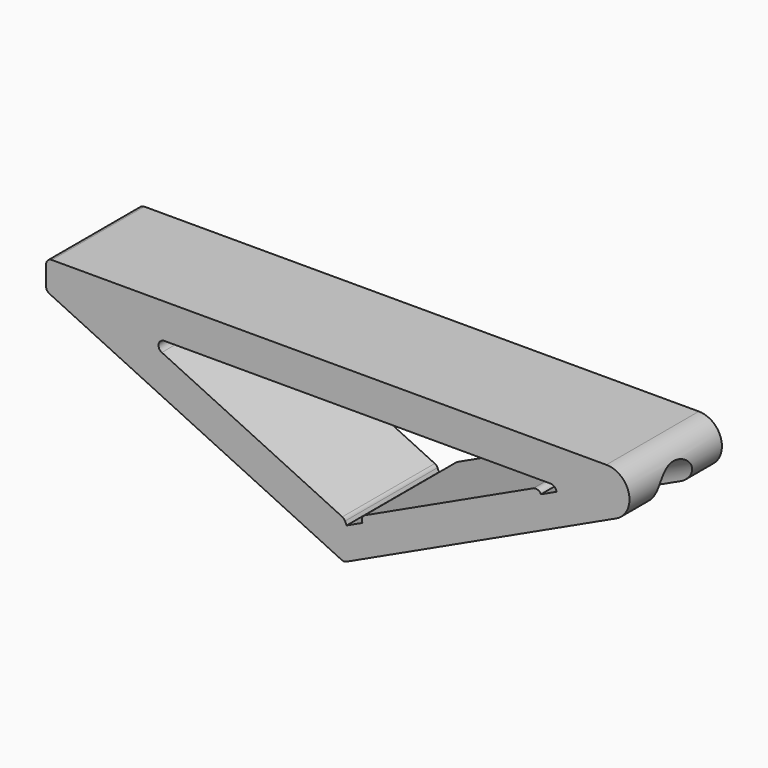
from build123d import *

# Parameters (mm, degrees)
F1_DEPTH  = 50
F3_R      = 1
F4_R      = 4
F5_R      = 4
F6_DEPTH  = 116.6842043143
F8_DEPTH  = 50.0010001
F9_R      = 0.99999
F10_DEPTH = 30


# Not quite as in the source:
# - a fillet or chamfer is up to 0.001 mm smaller than in the source, because OpenCascade refuses the exact size


with BuildPart() as f1:
    # F0 (on Front) → F1 (new body)
    with BuildSketch(Plane.XZ):
        Polygon((-63.4415450926, -29.5832783218), (0, 0), (-115, 0), (-115, -5), align=None)
    extrude(amount=F1_DEPTH)

    # F3
    f3_edges = [f1.edges().sort_by_distance(p)[0] for p in [
        (-63.441545, -25, -29.583278),
        (-115, -25, -5),
        (-115, -25, 0),
    ]]
    fillet(f3_edges, radius=F3_R)

    # F4
    f4_edges = [f1.edges().sort_by_distance(p)[0] for p in [
        (0, -25, 0),
    ]]
    fillet(f4_edges, radius=F4_R)

    # F5 (on face) → F6 (cut, through all)
    with BuildSketch(Plane(origin=(0, 0, 0), x_dir=(0, 1, 0), z_dir=(0.906307787, 0, 0.4226182617))):
        with Locations((-40, 0)):
            Circle(F5_R)
    extrude(amount=-F6_DEPTH, mode=Mode.SUBTRACT)

    # F7 (on Front) → F8 (cut, through all)
    with BuildSketch(Plane.XZ):
        Polygon((-27.064251022, -6), (-98.9616948614, -6), (-63.4130640807, -22.9497298941), (-62.990445819, -23.8560376812), (-60.2715224579, -22.588182896), (-60.6941407196, -21.6818751089), (-29.7831743831, -7.2678547852), (-29.3605561213, -8.1741625723), (-26.6416327602, -6.906307787), align=None)
    extrude(amount=F8_DEPTH, mode=Mode.SUBTRACT)

    # F9 (radius 1 in the source; OpenCascade refuses exactly that, so slightly less here)
    f9_edges = [f1.edges().sort_by_distance(p)[0] for p in [
        (-98.961695, -25, -6),
        (-60.694141, -25, -21.681875),
        (-29.783174, -25, -7.267855),
        (-27.064251, -25, -6),
        (-63.413064, -25, -22.94973),
    ]]
    fillet(f9_edges, radius=F9_R)

    # F0 (on Front) → F10 (cut)
    with BuildSketch(Plane.XZ):
        Polygon((-63.4415450926, -29.5832783218), (0, 0), (-115, 0), (-115, -5), align=None)
    extrude(amount=F10_DEPTH, mode=Mode.SUBTRACT)


solid = f1.part
